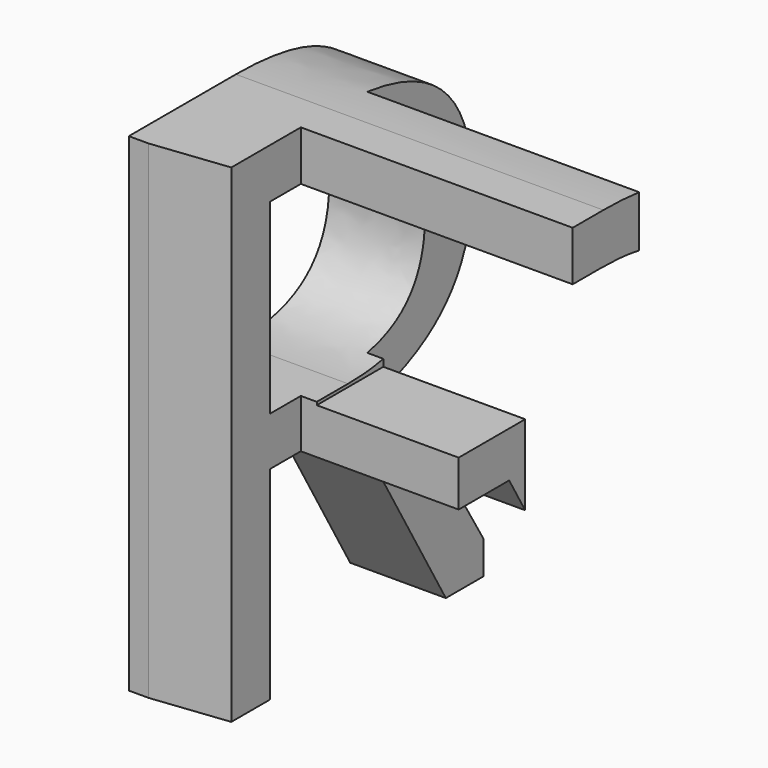
from build123d import *

# Parameters (mm, degrees)
F0_TEXT_SIZE = 206.5208326611
F1_DEPTH     = 111
F3_DEPTH     = 333
F6_DEPTH     = 292.2068536282


# Not quite as in the source:
# - Text() gives the source's letters only with a copy of the font that has no kerning and outlines rounded to 1/6400 em; it was checked with that copy


with BuildPart() as f1:
    # F0 (on Right) → F1 (new body)
    with BuildSketch(Plane.YZ):
        with Locations((-74.2397606373, -75.1147344708)):
            Text('R', F0_TEXT_SIZE, font='Open Sans', text_align=(TextAlign.LEFT, TextAlign.BOTTOM))
    extrude(amount=F1_DEPTH)

    # F2 (on face) → F3 (intersect)
    with BuildSketch(Plane.XZ.offset(53.9749039324)):
        Polygon((0, 72.3217787211), (0, -75.1147344708), (33.6987823248, -75.1147344708), (33.6987823248, -30.3394682705), (76.5611082315, -30.3394682705), (76.5611082315, 0), (33.6987823248, 0), (33.6987823248, 37.6816540956), (111, 37.6816540956), (111, 72.3217787211), align=None)
    extrude(amount=-F3_DEPTH, mode=Mode.INTERSECT)

    # F5 (on face) → F6 (intersect)
    with BuildSketch(Plane.XY.offset(72.3217787211)):
        Polygon((0, 43.7807589769), (0, -54.6587854624), (28.8827344775, -51.3631701469), (28.8827344775, -25.1220650971), (113.6668249965, -25.1220650971), (113.6668249965, 0), (28.8827344775, 0), (28.8827344775, 43.7807589769), align=None)
    extrude(amount=-F6_DEPTH, mode=Mode.INTERSECT)


solid = f1.part
